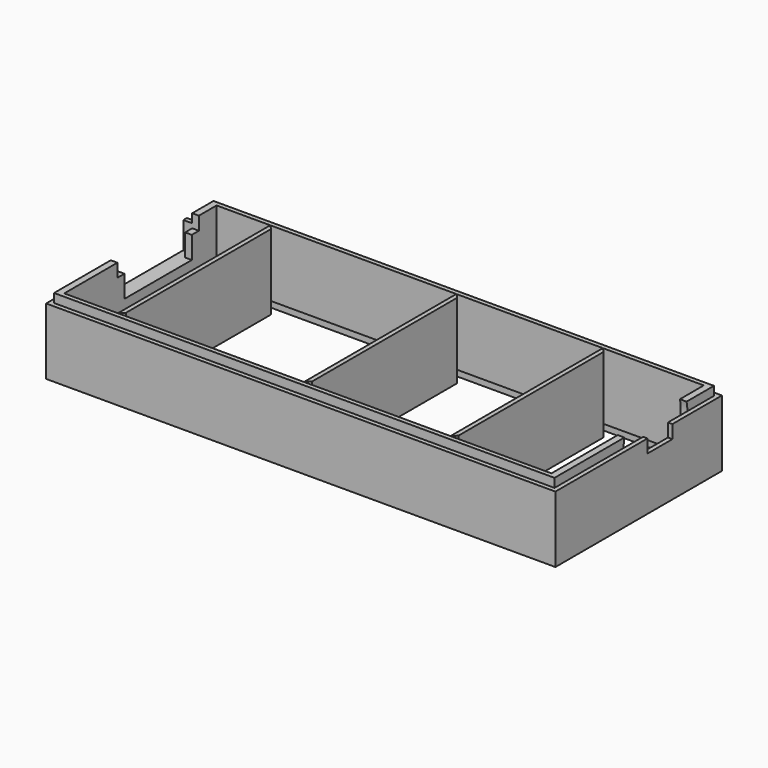
from build123d import *

# Parameters (mm, degrees)
F0_W      = 115
F0_H      = 47
F0_W_2    = 112
F0_H_2    = 45
F1_DEPTH  = 15
F3_W      = 113
F3_H      = 45
F3_W_2    = 110
F3_H_2    = 43
F4_DEPTH  = 15
F5_W      = 7
F5_H      = 2
F5_H_2    = 3
F6_DEPTH  = 25
F8_DEPTH  = 1.5
F9_W      = 2
F9_H      = 3
F9_W_2    = 19
F9_H_2    = 5
F10_DEPTH = 25
F12_DEPTH = 1
F13_DEPTH = 1
F15_DEPTH = 17


with BuildPart() as f1:
    # F0 (on Top) → F1 (new body)
    with BuildSketch(Plane.XY):
        Rectangle(F0_W, F0_H)
        Rectangle(F0_W_2, F0_H_2, mode=Mode.SUBTRACT)
    extrude(amount=F1_DEPTH)

    # F3 (on offset) → F4 (join)
    with BuildSketch(Plane.XY.offset(2)):
        Rectangle(F3_W, F3_H)
        Rectangle(F3_W_2, F3_H_2, mode=Mode.SUBTRACT)
    extrude(amount=F4_DEPTH)

    # F5 (on face) → F6 (cut)
    with BuildSketch(Plane.YZ.offset(57.5)):
        with Locations((6, 16)):
            Rectangle(F5_W, F5_H)
        with Locations((6, 13.5)):
            Rectangle(F5_W, F5_H_2)
    extrude(amount=-F6_DEPTH, mode=Mode.SUBTRACT)

    # F7 (on face) → F8 (cut)
    with BuildSketch(Plane(origin=(55, 0, 0), x_dir=(0, -1, 0), z_dir=(-1, 0, 0))):
        with BuildLine():
            ThreePointArc((-14.7749643874, 17), (-7.0063102189, 6.0564358479), (3, 15))
            ThreePointArc((3, 15), (2.9435641521, 16.0063102189), (2.7749643874, 17))
            Line((2.7749643874, 17), (-2.5, 17))
            Line((-2.5, 17), (-2.5, 12))
            Line((-2.5, 12), (-9.5, 12))
            Line((-9.5, 12), (-9.5, 17))
            Line((-9.5, 17), (-14.7749643874, 17))
        make_face()
        with BuildLine():
            Line((-2.5, 17), (2.7749643874, 17))
            ThreePointArc((2.7749643874, 17), (-6, 24), (-14.7749643874, 17))
            Line((-14.7749643874, 17), (-9.5, 17))
            Line((-9.5, 17), (-9.5, 12))
            Line((-9.5, 12), (-2.5, 12))
            Line((-2.5, 12), (-2.5, 17))
        make_face()
    extrude(amount=-F8_DEPTH, mode=Mode.SUBTRACT)

    # F9 (on face) → F10 (cut)
    with BuildSketch(Plane.YZ.offset(-55)):
        with Locations((-5.5, 15.5)):
            Rectangle(F9_W, F9_H)
        with Locations((5, 11.5)):
            Rectangle(F9_W_2, F9_H_2)
        with Locations((15.5, 15.5)):
            Rectangle(F9_W, F9_H)
        with Locations((5, 15.5)):
            Rectangle(F9_W_2, F9_H)
    extrude(amount=-F10_DEPTH, mode=Mode.SUBTRACT)

    # F11 (on face) → F12 (join)
    with BuildSketch(Plane(origin=(-57.5, 0, 0), x_dir=(0, -1, 0), z_dir=(-1, 0, 0))):
        Polygon((-16.5, 15), (-17.5, 15), (-17.5, 8), (7.5, 8), (7.5, 15), (6.5, 15), (6.5, 14), (6.5, 9), (4.5, 9), (-14.5, 9), (-16.5, 9), (-16.5, 14), align=None)
    extrude(amount=F12_DEPTH)

    # F13 (cut): faces of the model
    f13_faces = [f1.faces().sort_by_distance(p)[0] for p in [
        (-57.5, 15.5, 11.5),
        (-57.5, -5.5, 11.5),
    ]]
    extrude(f13_faces, amount=-F13_DEPTH, mode=Mode.SUBTRACT)


with BuildPart() as f15:
    # F14 (on Top) → F15 (new body)
    with BuildSketch(Plane.XY):
        Polygon((-41.8804898377, 20.5), (-42.8804898377, 21.5), (-42.8804898377, -21.5), (-41.8804898377, -20.5), align=None)
    extrude(amount=F15_DEPTH)


with BuildPart() as f15b:
    # F14 (on Top) → F15, piece 2 (new body)
    with BuildSketch(Plane.XY):
        Polygon((0.1358912904, 20.5), (-0.8641087096, 21.5), (-0.8641087096, -21.449737452), (0.1358912904, -20.5), align=None)
    extrude(amount=F15_DEPTH)


with BuildPart() as f15c:
    # F14 (on Top) → F15, piece 3 (new body)
    with BuildSketch(Plane.XY):
        Polygon((33.2106517851, 20.5), (32.2106517851, 21.5), (32.2106517851, -21.5), (33.2106517851, -20.5), align=None)
    extrude(amount=F15_DEPTH)


solid = Compound([f1.part, f15.part, f15b.part, f15c.part])
